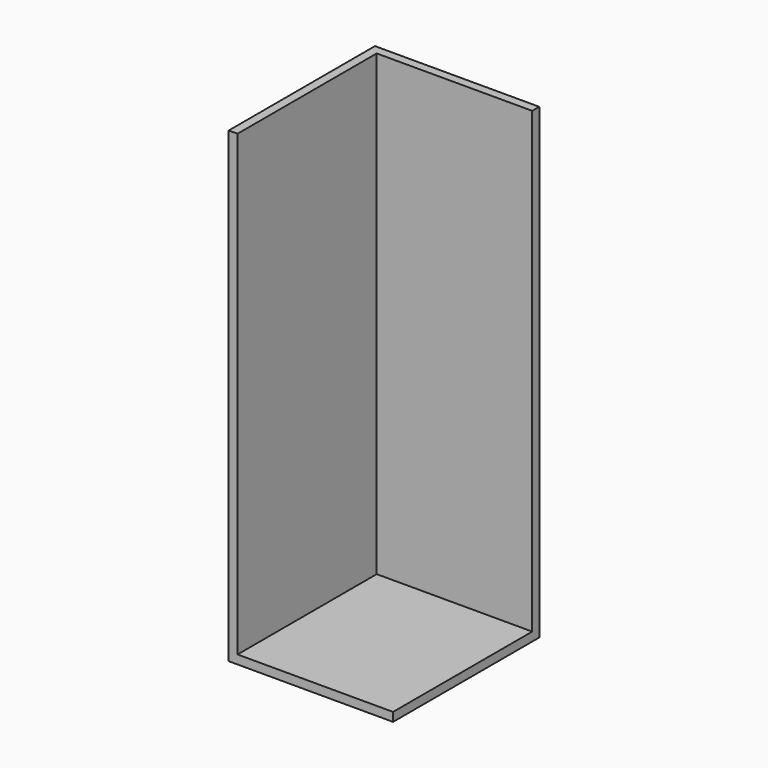
from build123d import *

# Parameters (mm, degrees)
F0_W     = 47.3500564694
F0_H     = 52.66610533
F1_DEPTH = 134.6403062344
F2_T     = -2.54


# Not quite as in the source:
# - a feature of the source that left no trace in its solid (it failed there, or was rolled back) is left out


with BuildPart() as f1:
    # F0 (on Top) → F1 (new body)
    with BuildSketch(Plane.XY):
        with Locations((23.6750282347, 26.333052665)):
            Rectangle(F0_W, F0_H)
    extrude(amount=F1_DEPTH)

    # F2
    f2_openings = [f1.faces().sort_by_distance(p)[0] for p in [
        (23.675028, 0, 67.320153),
        (47.350056, 26.333053, 67.320153),
        (23.675028, 26.333053, 134.640306),
    ]]
    offset(amount=F2_T, openings=f2_openings)


solid = f1.part
